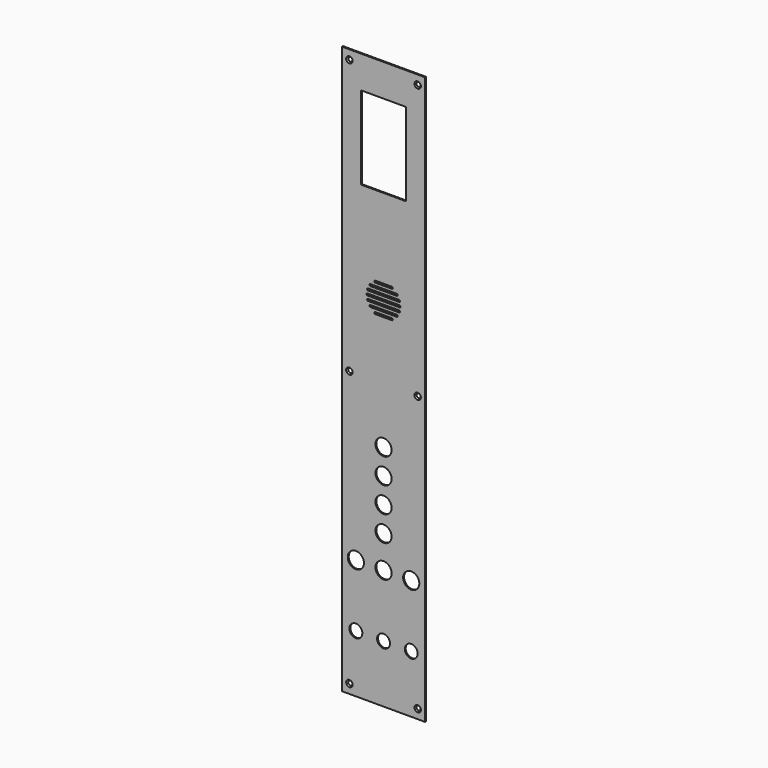
from build123d import *

# Parameters (mm, degrees)
F0_W     = 180
F0_H     = 1230
F0_R     = 3
F0_R_2   = 14
F0_R_3   = 17.5
F0_W_2   = 98
F0_H_2   = 180
F1_DEPTH = 2.5


# Not quite as in the source:
# - a fillet or chamfer that OpenCascade refuses, or shapes differently, is made with other operations: its cross-section is extruded or revolved along the edge and cut away or added
# - the program builds the solid bodies; features that only make, move or delete a surface that nothing else refers to are left out


with BuildPart() as f1:
    # F0 (on Front) → F1 (new body)
    with BuildSketch(Plane.XZ):
        with Locations((-49, -0.441852957)):
            Rectangle(F0_W, F0_H)
        with Locations((-123, -595.441852957)):
            Circle(F0_R, mode=Mode.SUBTRACT)
        with Locations((-109, -490.441852957)):
            Circle(F0_R_2, mode=Mode.SUBTRACT)
        with Locations((-109, -355.441852957)):
            Circle(F0_R_3, mode=Mode.SUBTRACT)
        with Locations((-49, -490.441852957)):
            Circle(F0_R_2, mode=Mode.SUBTRACT)
        with Locations((-49, -355.441852957)):
            Circle(F0_R_3, mode=Mode.SUBTRACT)
        with Locations((11, -490.441852957)):
            Circle(F0_R_2, mode=Mode.SUBTRACT)
        with Locations((25, -595.441852957)):
            Circle(F0_R, mode=Mode.SUBTRACT)
        with Locations((11, -355.441852957)):
            Circle(F0_R_3, mode=Mode.SUBTRACT)
        with Locations((-49, -285.441852957)):
            Circle(F0_R_3, mode=Mode.SUBTRACT)
        with Locations((-49, -230.441852957)):
            Circle(F0_R_3, mode=Mode.SUBTRACT)
        with Locations((-49, -175.441852957)):
            Circle(F0_R_3, mode=Mode.SUBTRACT)
        with Locations((-49, -120.441852957)):
            Circle(F0_R_3, mode=Mode.SUBTRACT)
        with Locations((-123, 0.558147043)):
            Circle(F0_R, mode=Mode.SUBTRACT)
        with BuildLine():
            Line((-30.9722436227, 127.558147043), (-67.0277563773, 127.558147043))
            ThreePointArc((-67.0277563773, 127.558147043), (-69.0277563773, 129.558147043), (-67.0277563773, 131.558147043))
            Line((-67.0277563773, 131.558147043), (-30.9722436227, 131.558147043))
            ThreePointArc((-30.9722436227, 131.558147043), (-28.9722436227, 129.558147043), (-30.9722436227, 127.558147043))
        make_face(mode=Mode.SUBTRACT)
        with BuildLine():
            Line((-20.2771867673, 137.558147043), (-77.7228132327, 137.558147043))
            ThreePointArc((-77.7228132327, 137.558147043), (-79.7228132327, 139.558147043), (-77.7228132327, 141.558147043))
            Line((-77.7228132327, 141.558147043), (-20.2771867673, 141.558147043))
            ThreePointArc((-20.2771867673, 141.558147043), (-18.2771867673, 139.558147043), (-20.2771867673, 137.558147043))
        make_face(mode=Mode.SUBTRACT)
        with BuildLine():
            Line((-15.4589803375, 147.558147043), (-82.5410196625, 147.558147043))
            ThreePointArc((-82.5410196625, 147.558147043), (-84.5410196625, 149.558147043), (-82.5410196625, 151.558147043))
            Line((-82.5410196625, 151.558147043), (-15.4589803375, 151.558147043))
            ThreePointArc((-15.4589803375, 151.558147043), (-13.4589803375, 149.558147043), (-15.4589803375, 147.558147043))
        make_face(mode=Mode.SUBTRACT)
        with BuildLine():
            Line((-15.4589803375, 167.558147043), (-82.5410196625, 167.558147043))
            ThreePointArc((-82.5410196625, 167.558147043), (-84.5410196625, 169.558147043), (-82.5410196625, 171.558147043))
            Line((-82.5410196625, 171.558147043), (-15.4589803375, 171.558147043))
            ThreePointArc((-15.4589803375, 171.558147043), (-13.4589803375, 169.558147043), (-15.4589803375, 167.558147043))
        make_face(mode=Mode.SUBTRACT)
        with BuildLine():
            Line((-20.2771867673, 177.558147043), (-77.7228132327, 177.558147043))
            ThreePointArc((-77.7228132327, 177.558147043), (-79.7228132327, 179.558147043), (-77.7228132327, 181.558147043))
            Line((-77.7228132327, 181.558147043), (-20.2771867673, 181.558147043))
            ThreePointArc((-20.2771867673, 181.558147043), (-18.2771867673, 179.558147043), (-20.2771867673, 177.558147043))
        make_face(mode=Mode.SUBTRACT)
        with BuildLine():
            Line((-30.9722436227, 187.558147043), (-67.0277563773, 187.558147043))
            ThreePointArc((-67.0277563773, 187.558147043), (-69.0277563773, 189.558147043), (-67.0277563773, 191.558147043))
            Line((-67.0277563773, 191.558147043), (-30.9722436227, 191.558147043))
            ThreePointArc((-30.9722436227, 191.558147043), (-28.9722436227, 189.558147043), (-30.9722436227, 187.558147043))
        make_face(mode=Mode.SUBTRACT)
        with Locations((-123, 594.558147043)):
            Circle(F0_R, mode=Mode.SUBTRACT)
        with BuildLine():
            Line((-14, 157.558147043), (-84, 157.558147043))
            ThreePointArc((-84, 157.558147043), (-86, 159.558147043), (-84, 161.558147043))
            Line((-84, 161.558147043), (-14, 161.558147043))
            ThreePointArc((-14, 161.558147043), (-12, 159.558147043), (-14, 157.558147043))
        make_face(mode=Mode.SUBTRACT)
        with Locations((25, 0.558147043)):
            Circle(F0_R, mode=Mode.SUBTRACT)
        with Locations((-49, 454.558147043)):
            Rectangle(F0_W_2, F0_H_2, mode=Mode.SUBTRACT)
        with Locations((25, 594.558147043)):
            Circle(F0_R, mode=Mode.SUBTRACT)
    extrude(amount=F1_DEPTH)

    # F2: chamfer of 4 on 6 edges, made by hand

    # F2_s1 → F2_t2 (revolve, cut)
    with BuildSketch(Plane.XY.offset(-595.441852957)):
        Polygon((28, 1.5), (32, -2.5), (28, -2.5), align=None)
    revolve(axis=Axis((25, -2.5, -595.441852957), (0, -1, 0)), mode=Mode.SUBTRACT)

    # F2_s3 → F2_t4 (revolve, cut)
    with BuildSketch(Plane.XY.offset(-595.441852957)):
        Polygon((-120, 1.5), (-116, -2.5), (-120, -2.5), align=None)
    revolve(axis=Axis((-123, -2.5, -595.441852957), (0, -1, 0)), mode=Mode.SUBTRACT)

    # F2_s5 → F2_t6 (revolve, cut)
    with BuildSketch(Plane.XY.offset(0.558147043)):
        Polygon((-120, 1.5), (-116, -2.5), (-120, -2.5), align=None)
    revolve(axis=Axis((-123, -2.5, 0.558147043), (0, -1, 0)), mode=Mode.SUBTRACT)

    # F2_s7 → F2_t8 (revolve, cut)
    with BuildSketch(Plane.XY.offset(0.558147043)):
        Polygon((28, 1.5), (32, -2.5), (28, -2.5), align=None)
    revolve(axis=Axis((25, -2.5, 0.558147043), (0, -1, 0)), mode=Mode.SUBTRACT)

    # F2_s9 → F2_t10 (revolve, cut)
    with BuildSketch(Plane.XY.offset(594.558147043)):
        Polygon((28, 1.5), (32, -2.5), (28, -2.5), align=None)
    revolve(axis=Axis((25, -2.5, 594.558147043), (0, -1, 0)), mode=Mode.SUBTRACT)

    # F2_s11 → F2_t12 (revolve, cut)
    with BuildSketch(Plane.XY.offset(594.558147043)):
        Polygon((-120, 1.5), (-116, -2.5), (-120, -2.5), align=None)
    revolve(axis=Axis((-123, -2.5, 594.558147043), (0, -1, 0)), mode=Mode.SUBTRACT)


solid = f1.part
